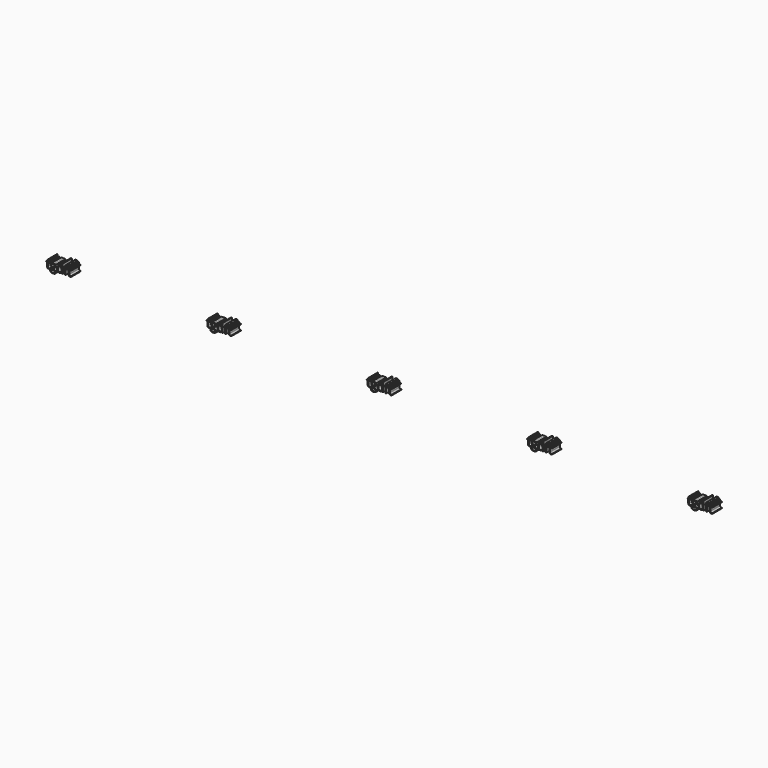
from build123d import *

# Parameters (mm, degrees)
F0_TEXT_SIZE = 24.1240383022
F1_DEPTH     = 25


# Not quite as in the source:
# - Text() gives the source's letters only with a copy of the font that has no kerning and outlines rounded to 1/6400 em; it was checked with that copy


with BuildPart() as f1:
    # F0 (on Front) → F1 (new body)
    with BuildSketch(Plane.XZ):
        with Locations((282.0816259919, 0)):
            Text('tgdft                                             tgdft                                             tgdft                                             tgdft                                             tgdft', F0_TEXT_SIZE, font='Open Sans', text_align=(TextAlign.LEFT, TextAlign.BOTTOM))
    extrude(amount=F1_DEPTH)


solid = f1.part
